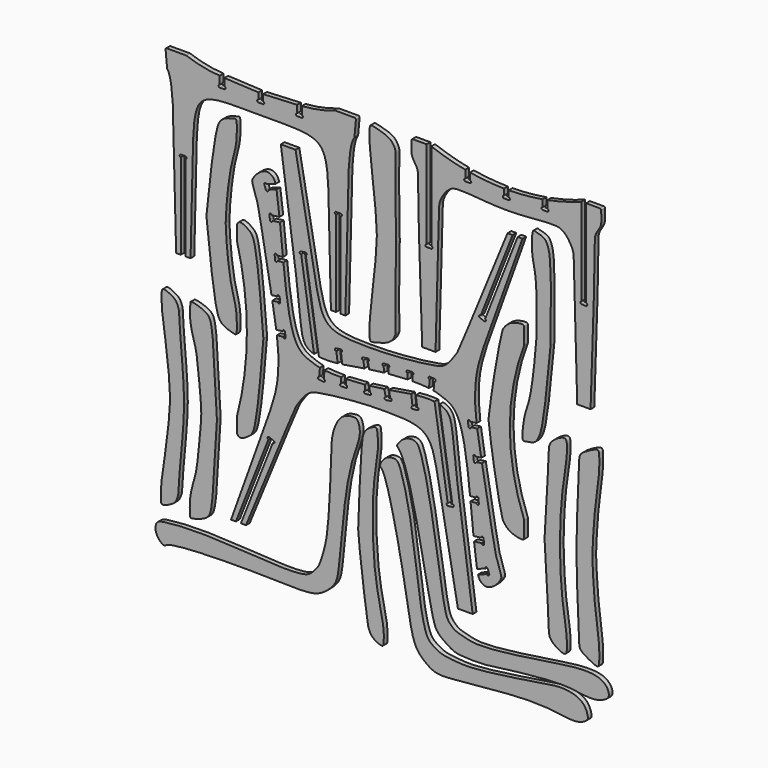
from build123d import *

# Parameters (mm, degrees)
F1_DEPTH = 11.90625
F3_DEPTH = 11.90625
F5_DEPTH = 11.90625
F7_DEPTH = 11.90625


with BuildPart() as f1:
    # F0 (on Front) → F1 (new body)
    with BuildSketch(Plane.XZ):
        with BuildLine():
            Line((-81.6249251366, 184.9817527294), (-81.6249251366, 205.2300572395))
            ThreePointArc((-81.6249251366, 205.2300572395), (-124.8707299183, 211.0284592013), (-166.8653927493, 222.8719971122))
            Line((-166.8653927493, 222.8719971122), (-216.4043151029, 222.8719971122))
            ThreePointArc((-216.4043151029, 222.8719971122), (-218.7506863203, 221.8359611396), (-219.5657662077, 219.4039921424))
            Line((-219.5657662077, 219.4039921424), (-215.716868639, 177.8753399849))
            add(Edge.make_bspline(
                [(-201.2570202351, 103.3167913556), (-203.5053147842, 133.6572504695), (-205.7536093334, 163.9977095834), (-215.716868639, 177.8753399849)],
                knots=[0, 0, 0, 0, 0.6286084073, 0.6286084073, 0.6286084073, 0.6286084073], degree=3))
            Line((-201.2570202351, 103.3167913556), (-192.6272958517, -229.0771717804))
            Line((-192.6272958517, -229.0771717804), (-180.7148461342, -228.9787826776))
            Line((-180.7148461342, -228.9787826776), (-180.7148461342, -10.1681035912))
            ThreePointArc((-180.7148461342, -10.1681035912), (-183.8898461342, -6.9931035912), (-180.7148461342, -3.8181035912))
            Line((-180.7148461342, -3.8181035912), (-168.8085961342, -3.8181035912))
            ThreePointArc((-168.8085961342, -3.8181035912), (-165.6335961342, -6.9931035912), (-168.8085961342, -10.1681035912))
            Line((-168.8085961342, -10.1681035912), (-168.8085961342, -228.8804447805))
            Line((-168.8085961342, -228.8804447805), (-155.8824628592, -228.7736833096))
            Line((-155.8824628592, -228.7736833096), (-149.3858247995, 40.4817350209))
            add(Edge.make_bspline(
                [(-149.3858247995, 40.4817350209), (-147.4859416485, 69.7398781776), (-146.2123086991, 156.4636002304), (-66.5898651674, 150.1531891202), (23.0572682768, 150.2735537717)],
                knots=[0, 0, 0, 0, 0.4228498511, 0.9834705051, 0.9834705051, 0.9834705051, 0.9834705051], degree=3))
            add(Edge.make_bspline(
                [(195.5003613532, 40.4817350209), (193.6004782021, 69.7398781776), (192.3268452527, 156.4636002304), (112.704401721, 150.1531891202), (23.0572682768, 150.2735537717)],
                knots=[0, 0, 0, 0, 0.4228498511, 0.9834705051, 0.9834705051, 0.9834705051, 0.9834705051], degree=3))
            Line((195.5003613532, 40.4817350209), (201.9969994128, -228.7736833096))
            Line((201.9969994128, -228.7736833096), (214.9231326878, -228.8804447805))
            Line((214.9231326878, -228.8804447805), (214.9231326878, -10.1681035912))
            ThreePointArc((214.9231326878, -10.1681035912), (211.7481326878, -6.9931035912), (214.9231326878, -3.8181035912))
            Line((214.9231326878, -3.8181035912), (226.8293826878, -3.8181035912))
            ThreePointArc((226.8293826878, -3.8181035912), (230.0043826878, -6.9931035912), (226.8293826878, -10.1681035912))
            Line((226.8293826878, -10.1681035912), (226.8293826878, -228.9787826776))
            Line((226.8293826878, -228.9787826776), (238.7418324053, -229.0771717804))
            Line((238.7418324053, -229.0771717804), (247.3715567887, 103.3167913556))
            add(Edge.make_bspline(
                [(247.3715567887, 103.3167913556), (249.6198513379, 133.6572504695), (251.868145887, 163.9977095834), (261.8314051926, 177.8753399849)],
                knots=[0, 0, 0, 0, 0.6286084073, 0.6286084073, 0.6286084073, 0.6286084073], degree=3))
            Line((261.8314051926, 177.8753399849), (265.6803027613, 219.4039921424))
            ThreePointArc((265.6803027613, 219.4039921424), (264.8652228739, 221.8359611396), (262.5188516565, 222.8719971122))
            Line((262.5188516565, 222.8719971122), (212.9799293029, 222.8719971122))
            ThreePointArc((212.9799293029, 222.8719971122), (170.9852664719, 211.0284592013), (127.7394616902, 205.2300572395))
            Line((127.7394616902, 205.2300572395), (127.7394616902, 184.9817527294))
            ThreePointArc((127.7394616902, 184.9817527294), (130.9144616902, 181.8067527294), (127.7394616902, 178.6317527294))
            Line((127.7394616902, 178.6317527294), (115.8332116902, 178.6317527294))
            ThreePointArc((115.8332116902, 178.6317527294), (112.6582116902, 181.8067527294), (115.8332116902, 184.9817527294))
            Line((115.8332116902, 184.9817527294), (115.8332116902, 204.0726095438))
            Line((115.8332116902, 204.0726095438), (29.0103932768, 199.9165117741))
            Line((29.0103932768, 199.9165117741), (29.0103932768, 183.5399461746))
            ThreePointArc((29.0103932768, 183.5399461746), (32.1853932768, 180.3649461746), (29.0103932768, 177.1899461746))
            Line((29.0103932768, 177.1899461746), (23.0572682768, 177.1899461746))
            Line((23.0572682768, 177.1899461746), (17.1041432768, 177.1899461746))
            ThreePointArc((17.1041432768, 177.1899461746), (13.9291432768, 180.3649461746), (17.1041432768, 183.5399461746))
            Line((17.1041432768, 183.5399461746), (17.1041432768, 199.9165117741))
            Line((17.1041432768, 199.9165117741), (-69.7186751366, 204.0726095438))
            Line((-69.7186751366, 204.0726095438), (-69.7186751366, 184.9817527294))
            ThreePointArc((-69.7186751366, 184.9817527294), (-66.5436751366, 181.8067527294), (-69.7186751366, 178.6317527294))
            Line((-69.7186751366, 178.6317527294), (-81.6249251366, 178.6317527294))
            ThreePointArc((-81.6249251366, 178.6317527294), (-84.7999251366, 181.8067527294), (-81.6249251366, 184.9817527294))
        make_face()
    extrude(amount=F1_DEPTH)


with BuildPart() as f1b:
    # F0 (on Front) → F1, piece 2 (new body)
    with BuildSketch(Plane.XZ):
        with BuildLine():
            Line((753.9582689397, 197.8409755017), (753.9392547607, 177.9192579746))
            ThreePointArc((753.9392547607, 177.9192579746), (757.1142547607, 174.7442579746), (753.9392547607, 171.5692579746))
            Line((753.9392547607, 171.5692579746), (742.0330047607, 171.5692579746))
            ThreePointArc((742.0330047607, 171.5692579746), (738.8580047607, 174.7442579746), (742.0330047607, 177.9192579746))
            Line((742.0330047607, 177.9192579746), (742.0330047607, 195.6590753576))
            ThreePointArc((742.0330047607, 195.6590753576), (698.8370899175, 189.9852566287), (655.3285871628, 187.7292721077))
            Line((655.3285871628, 187.7292721077), (655.3285871628, 171.9064457408))
            ThreePointArc((655.3285871628, 171.9064457408), (658.5035871628, 168.7314457408), (655.3285871628, 165.5564457408))
            Line((655.3285871628, 165.5564457408), (649.375430584, 165.5564457408))
            Line((649.375430584, 165.5564457408), (643.4222740051, 165.5564457408))
            ThreePointArc((643.4222740051, 165.5564457408), (640.2472740051, 168.7314457408), (643.4222740051, 171.9064457408))
            Line((643.4222740051, 171.9064457408), (643.4222740051, 187.7292721077))
            ThreePointArc((643.4222740051, 187.7292721077), (599.9137712504, 189.9852566287), (556.7178564072, 195.6590753576))
            Line((556.7178564072, 195.6590753576), (556.7178564072, 177.9192579746))
            ThreePointArc((556.7178564072, 177.9192579746), (559.8928564072, 174.7442579746), (556.7178564072, 171.5692579746))
            Line((556.7178564072, 171.5692579746), (544.8116064072, 171.5692579746))
            ThreePointArc((544.8116064072, 171.5692579746), (541.6366064072, 174.7442579746), (544.8116064072, 177.9192579746))
            Line((544.8116064072, 177.9192579746), (544.7925922282, 197.8409755017))
            ThreePointArc((544.7925922282, 197.8409755017), (500.8902250493, 208.2467794905), (457.9821969142, 222.1966799246))
            Line((457.9821969142, 222.1966799246), (457.8196128837, -1.4435426646))
            ThreePointArc((457.8196128837, -1.4435426646), (460.9842648937, -4.6208339943), (457.8149965181, -7.7935206322))
            Line((457.8149965181, -7.7935206322), (445.9087465181, -7.7935218998))
            ThreePointArc((445.9087465181, -7.7935218998), (442.7744985153, -4.5708815102), (446.0045408796, -1.4442622579))
            Line((446.0045408796, -1.4442622579), (446.0045408796, 222.833275795))
            Line((446.0045408796, 222.833275795), (410.7614188056, 222.833275795))
            ThreePointArc((410.7614188056, 222.833275795), (408.5663096829, 221.9522071234), (407.5894946571, 219.7979976465))
            add(Edge.make_bspline(
                [(407.5894946571, 219.7979976465), (407.0855216225, 208.3569508739), (406.4295588438, 189.5758183878), (411.4862805096, 177.3822155111), (425.682188243, 158.4107209843), (422.6201017336, 109.1856224555), (429.5663710054, -88.2138828921), (434.7653226852, -235.9580099583)],
                knots=[0.0119439068, 0.0119439068, 0.0119439068, 0.0119439068, 0.1472174846, 0.2400583983, 0.3538051352, 0.5163539238, 1, 1, 1, 1], degree=3))
            Line((434.7653226852, -235.9580099583), (468.7381820679, -235.9580099583))
            add(Edge.make_bspline(
                [(468.7381820679, -235.9580099583), (472.4303966062, -104.6167901897), (477.3449907849, 70.2075022277), (477.7680787876, 108.7569713641), (502.1370780301, 143.5053595047), (529.180974636, 149.9698487576), (609.7624332079, 141.4228850822), (638.3718253047, 141.2618428968), (649.3754305839, 141.2687947189)],
                knots=[0, 0, 0, 0, 0.3522357263, 0.4688502339, 0.5878047938, 0.6920991895, 0.8721155501, 0.9906857663, 0.9906857663, 0.9906857663, 0.9906857663], degree=3))
            add(Edge.make_bspline(
                [(830.0126791, -235.9580099583), (826.3204645618, -104.6167901897), (821.405870383, 70.2075022277), (820.9827823803, 108.7569713641), (796.6137831378, 143.5053595047), (769.5698865319, 149.9698487576), (688.98842796, 141.4228850822), (660.3790358632, 141.2618428968), (649.3754305839, 141.2687947189)],
                knots=[0, 0, 0, 0, 0.3522357263, 0.4688502339, 0.5878047938, 0.6920991895, 0.8721155501, 0.9906857663, 0.9906857663, 0.9906857663, 0.9906857663], degree=3))
            Line((830.0126791, -235.9580099583), (863.9855384827, -235.9580099583))
            add(Edge.make_bspline(
                [(891.1613665108, 219.7979976465), (891.6653395454, 208.3569508739), (892.3213023241, 189.5758183878), (887.2645806583, 177.3822155111), (873.0686729249, 158.4107209843), (876.1307594343, 109.1856224555), (869.1844901625, -88.2138828921), (863.9855384827, -235.9580099583)],
                knots=[0.0119439068, 0.0119439068, 0.0119439068, 0.0119439068, 0.1472174846, 0.2400583983, 0.3538051352, 0.5163539238, 1, 1, 1, 1], degree=3))
            ThreePointArc((891.1613665108, 219.7979976465), (890.184551485, 221.9522071234), (887.9894423623, 222.833275795))
            Line((887.9894423623, 222.833275795), (852.7463202883, 222.833275795))
            Line((852.7463202883, 222.833275795), (852.7463202883, -1.4442622579))
            ThreePointArc((852.7463202883, -1.4442622579), (855.9763626526, -4.5708815102), (852.8421146498, -7.7935218998))
            Line((852.8421146498, -7.7935218998), (840.9358646498, -7.7935206322))
            ThreePointArc((840.9358646498, -7.7935206322), (837.7665962742, -4.6208339943), (840.9312482842, -1.4435426646))
            Line((840.9312482842, -1.4435426646), (840.7686642537, 222.1966799246))
            ThreePointArc((840.7686642537, 222.1966799246), (797.8606361186, 208.2467794905), (753.9582689397, 197.8409755017))
        make_face()
    extrude(amount=F1_DEPTH)


with BuildPart() as f3:
    # F2 (on Front) → F3 (new body)
    with BuildSketch(Plane.XZ):
        with BuildLine():
            add(Edge.make_bspline(
                [(566.8695082514, -629.2812363074), (569.5853295665, -654.3702688331), (572.1095143597, -675.1237511334), (574.4261674133, -688.4633543022)],
                knots=[0.5041739496, 0.5041739496, 0.5041739496, 0.5041739496, 0.5323722078, 0.5323722078, 0.5323722078, 0.5323722078], degree=3))
            Line((574.4261674133, -688.4633543022), (595.5900230834, -680.886998067))
            ThreePointArc((595.5900230834, -680.886998067), (597.509152839, -676.827664257), (601.568486649, -678.7467940126))
            Line((601.568486649, -678.7467940126), (605.581369251, -689.9564131981))
            ThreePointArc((605.581369251, -689.9564131981), (603.6622394954, -694.0157470081), (599.6029056854, -692.0966172525))
            Line((599.6029056854, -692.0966172525), (576.9251566248, -700.2149255691))
            add(Edge.make_bspline(
                [(576.9251566248, -700.2149255691), (577.9995338219, -704.1085984084), (580.5037674854, -710.1106761836), (586.6774372848, -717.4303434775), (600.064292499, -722.9901001137), (619.8937899939, -713.2743570691), (632.3782583366, -697.6701022409), (639.353554629, -686.8491619857), (623.0185314321, -652.1785312949), (612.0860881001, -584.9638273352), (595.1931225708, -492.5807100816), (587.236787797, -447.3290557083)],
                knots=[0.5426631517, 0.5426631517, 0.5426631517, 0.5426631517, 0.5556846822, 0.5709687245, 0.5884954803, 0.6108677295, 0.6326246328, 0.6485941027, 0.6762818943, 0.7187139825, 0.7710183017, 0.7710183017, 0.7710183017, 0.7710183017], degree=3))
            Line((587.236787797, -447.3290557084), (572.6997915784, -449.1565687147))
            ThreePointArc((572.6997915784, -449.1565687147), (569.9456139325, -452.7027998824), (566.3993827648, -449.9486222365))
            Line((566.3993827648, -449.9486222365), (564.9142824113, -438.135355711))
            ThreePointArc((564.9142824113, -438.135355711), (567.6684600572, -434.5891245433), (571.2146912249, -437.3433021891))
            Line((571.2146912249, -437.3433021891), (585.1811060506, -435.5875196078))
            add(Edge.make_bspline(
                [(585.1811060506, -435.5875196079), (584.4323143041, -431.2907071066), (580.526436641, -408.7505367433), (577.1870397166, -388.6642774653), (575.0108794965, -373.3527850809)],
                knots=[0.775597785, 0.775597785, 0.775597785, 0.775597785, 0.7806933084, 0.8027679956, 0.8027679956, 0.8027679956, 0.8027679956], degree=3))
            Line((575.0108794965, -373.3527850808), (559.0072337667, -375.3646773782))
            ThreePointArc((559.0072337667, -375.3646773782), (556.2530561208, -378.9109085459), (552.706824953, -376.1567309001))
            Line((552.706824953, -376.1567309001), (551.2217245996, -364.3434643745))
            ThreePointArc((551.2217245996, -364.3434643745), (553.9759022455, -360.7972332068), (557.5221334132, -363.5514108527))
            Line((557.5221334132, -363.5514108527), (573.4188186259, -361.5529650564))
            add(Edge.make_bspline(
                [(573.4188186259, -361.5529650565), (571.541615983, -346.7842885987), (567.7068869039, -305.7710886357), (572.2446272444, -236.4022129148), (605.6116131937, -145.0539413696), (673.6225943328, 43.7902893513), (690.3986930847, 90.3371274471)],
                knots=[0.8085324624, 0.8085324624, 0.8085324624, 0.8085324624, 0.8305204676, 0.8732825465, 0.9238130436, 1, 1, 1, 1], degree=3))
            Line((690.3986930847, 90.3371274471), (677.9750958085, 90.3371274471))
            Line((677.9750958085, 90.3371274471), (595.1901786029, -120.6226050854))
            ThreePointArc((595.1901786029, -120.6226050854), (596.9859254868, -124.7380082405), (592.8705223316, -126.5337551243))
            Line((592.8705223316, -126.5337551243), (581.7871160086, -122.1843996156))
            ThreePointArc((581.7871160086, -122.1843996156), (579.9913691248, -118.0689964605), (584.1067722799, -116.2732495767))
            Line((584.1067722799, -116.2732495767), (665.1849133564, 90.3371274471))
            Line((665.1849133564, 90.3371274471), (652.2805280983, 90.3371274471))
            add(Edge.make_bspline(
                [(652.2805280983, 90.3371274471), (596.7992489646, -44.9195170026), (529.8230377107, -208.1994148996), (523.2153969383, -221.3143134207), (497.4125593379, -258.4004771389), (467.6212718132, -269.0955724434), (359.0838115877, -280.6103699551), (283.1255249355, -281.2402915833), (222.7475667298, -278.8147196555), (191.4119530649, -263.556681825), (172.6586255781, -230.6504371588), (157.6041323146, -145.7013190048), (129.7748164105, 4.8959686394), (111.855674535, 101.8647253513)],
                knots=[0, 0, 0, 0, 0.1855154705, 0.2239516381, 0.2883693718, 0.3471684711, 0.4532029351, 0.5467207513, 0.6247930511, 0.6828197717, 0.7416883994, 0.8336745957, 1, 1, 1, 1], degree=3))
            Line((111.855674535, 101.8647253513), (74.2674358189, 101.8647253513))
            add(Edge.make_bspline(
                [(74.2674358189, 101.8647253513), (78.8915198201, 69.5147677357), (83.5137174572, 37.1780070688), (87.9711113313, 5.7144869035)],
                knots=[0, 0, 0, 0, 0.0229430236, 0.0229430236, 0.0229430236, 0.0229430236], degree=3))
            add(Edge.make_bspline(
                [(87.9711113313, 5.7144869035), (100.6031911897, -83.4518983389), (119.6075895959, -221.5137269482), (125.5186145516, -299.1595751985), (134.8803023203, -330.0648259095), (149.5395161253, -338.7788583075), (158.9980423115, -341.3134779083)],
                knots=[0.0229430236, 0.0229430236, 0.0229430236, 0.0229430236, 0.0879626549, 0.1322113205, 0.1576764492, 0.1813971108, 0.1813971108, 0.1813971108, 0.1813971108], degree=3))
            Line((158.9980423115, -341.3134779083), (126.1187144879, -128.2851324575))
            ThreePointArc((126.1187144879, -128.2851324575), (122.4965658301, -125.6315897123), (125.1501085753, -122.0094410544))
            Line((125.1501085753, -122.0094410544), (136.917029956, -120.1933049683))
            ThreePointArc((136.917029956, -120.1933049683), (140.5391786138, -122.8468477135), (137.8856358686, -126.4689963713))
            Line((137.8856358686, -126.4689963713), (171.394359373, -343.5752573204))
            add(Edge.make_bspline(
                [(171.394359373, -343.5752573204), (184.8736689285, -345.1120254544), (201.6749889802, -344.5009932843), (218.5750232266, -342.6842309365), (219.1755757519, -342.6182161686)],
                knots=[0.1908558182, 0.1908558182, 0.1908558182, 0.1908558182, 0.2194262024, 0.2204785746, 0.2204785746, 0.2204785746, 0.2204785746], degree=3))
            Line((219.1755757519, -342.6182161686), (215.869193574, -316.3175195105))
            ThreePointArc((215.869193574, -316.3175195105), (212.3229624062, -313.5633418646), (215.0771400521, -310.0171106969))
            Line((215.0771400521, -310.0171106969), (226.8904065776, -308.5320103434))
            ThreePointArc((226.8904065776, -308.5320103434), (230.4366377453, -311.2861879893), (227.6824600995, -314.832419157))
            Line((227.6824600995, -314.832419157), (230.9906811714, -341.1477433423))
            add(Edge.make_bspline(
                [(230.9906811715, -341.1477433423), (249.07955335, -338.6582784106), (267.5544694031, -335.1362268397), (287.5048138783, -331.8922872279)],
                knots=[0.2273609107, 0.2273609107, 0.2273609107, 0.2273609107, 0.2588542647, 0.2588542647, 0.2588542647, 0.2588542647], degree=3))
            Line((287.5048138784, -331.8922872279), (284.5437138697, -314.7883116116))
            ThreePointArc((284.5437138697, -314.7883116116), (280.8736399921, -312.2014587489), (283.4604928548, -308.5313848714))
            Line((283.4604928548, -308.5313848714), (295.1922304928, -306.5003454685))
            ThreePointArc((295.1922304928, -306.5003454685), (298.8623043704, -309.0871983312), (296.2754515077, -312.7572722088))
            Line((296.2754515077, -312.7572722088), (299.2688604156, -330.0478712496))
            add(Edge.make_bspline(
                [(299.2688604156, -330.0478712496), (311.6334559032, -328.1866698123), (324.5238565238, -326.4939882328), (337.5390271034, -325.0741291087)],
                knots=[0.2649537217, 0.2649537217, 0.2649537217, 0.2649537217, 0.2839083997, 0.2839083997, 0.2839083997, 0.2839083997], degree=3))
            Line((337.5390271034, -325.0741291087), (336.3677488719, -310.9681260445))
            ThreePointArc((336.3677488719, -310.9681260445), (332.9409089755, -308.0667439041), (335.8422911159, -304.6399040078))
            Line((335.8422911159, -304.6399040078), (347.7077074349, -303.6546707153))
            ThreePointArc((347.7077074349, -303.6546707153), (351.1345473313, -306.5560528557), (348.2331651908, -309.9828927521))
            Line((348.2331651908, -309.9828927521), (349.3856222375, -323.8622274778))
            add(Edge.make_bspline(
                [(349.3856222375, -323.8622274778), (363.9828662923, -322.4699635009), (380.41617949, -321.3314170465), (396.1444916825, -320.8597404872), (397.8871803284, -320.8154072931)],
                knots=[0.2896480836, 0.2896480836, 0.2896480836, 0.2896480836, 0.3108436467, 0.313502856, 0.313502856, 0.313502856, 0.313502856], degree=3))
            Line((397.8871803284, -320.8154072931), (397.4540628227, -307.0115702828))
            ThreePointArc((397.4540628227, -307.0115702828), (394.1810528385, -303.9377037205), (397.2549194007, -300.6646937362))
            Line((397.2549194007, -300.6646937362), (409.1553129256, -300.2912998199))
            ThreePointArc((409.1553129256, -300.2912998199), (412.4283229099, -303.3651663822), (409.3544563476, -306.6381763665))
            Line((409.3544563476, -306.6381763665), (409.7937739849, -320.6396170431))
            add(Edge.make_bspline(
                [(409.793773985, -320.6396170431), (425.7267691669, -320.5793075671), (440.3219423663, -321.2493581383), (451.9999158307, -322.6158233251)],
                knots=[0.3196576333, 0.3196576333, 0.3196576333, 0.3196576333, 0.3448245133, 0.3448245133, 0.3448245133, 0.3448245133], degree=3))
            Line((451.9999158307, -322.6158233251), (453.8983790613, -302.3204325437))
            ThreePointArc((453.8983790613, -302.3204325437), (451.0328829105, -298.8635290436), (454.4897864107, -295.9980328927))
            Line((454.4897864107, -295.9980328927), (466.3442857563, -297.1069216728))
            ThreePointArc((466.3442857563, -297.1069216728), (469.2097819072, -300.563825173), (465.752878407, -303.4293213238))
            Line((465.752878407, -303.4293213238), (463.7880346946, -324.4343480869))
            add(Edge.make_bspline(
                [(463.7880346946, -324.4343480869), (471.9039207593, -326.0572697828), (487.0014775824, -331.2603228654), (536.9638470038, -348.6264520909), (549.6036944238, -459.5964349534), (556.7808309902, -530.3787318412)],
                knots=[0.3542148453, 0.3542148453, 0.3542148453, 0.3542148453, 0.3759368259, 0.4073734484, 0.4717986423, 0.4717986423, 0.4717986423, 0.4717986423], degree=3))
            Line((556.7808309902, -530.3787318412), (571.8823122062, -529.2545845291))
            ThreePointArc((571.8823122062, -529.2545845291), (574.8128584467, -525.8526514415), (578.2147915343, -528.7831976821))
            Line((578.2147915343, -528.7831976821), (579.0986418724, -540.6565964222))
            ThreePointArc((579.0986418724, -540.6565964222), (576.1680956319, -544.0585295097), (572.7661625443, -541.1279832692))
            Line((572.7661625443, -541.1279832692), (557.9763695577, -542.228928653))
            add(Edge.make_bspline(
                [(557.9763695577, -542.228928653), (560.6548814033, -568.8653653623), (563.2016059701, -594.6039142121), (565.6061929157, -617.4400881619)],
                knots=[0.4754072925, 0.4754072925, 0.4754072925, 0.4754072925, 0.4998482581, 0.4998482581, 0.4998482581, 0.4998482581], degree=3))
            Line((565.6061929158, -617.4400881619), (584.813059481, -615.0255041632))
            ThreePointArc((584.813059481, -615.0255041632), (587.5672371269, -611.4792729955), (591.1134682947, -614.2334506414))
            Line((591.1134682947, -614.2334506414), (592.5985686481, -626.0467171669))
            ThreePointArc((592.5985686481, -626.0467171669), (589.8443910022, -629.5929483346), (586.2981598345, -626.8387706887))
            Line((586.2981598345, -626.8387706887), (566.8695082514, -629.2812363074))
        make_face()
    extrude(amount=F3_DEPTH)


with BuildPart() as f3b:
    # F2 (on Front) → F3, piece 2 (new body)
    with BuildSketch(Plane.XZ):
        with BuildLine():
            Line((525.8545875549, -793.4511899948), (563.4428262711, -793.4511899948))
            add(Edge.make_bspline(
                [(563.4428262711, -793.4511899948), (558.8187422699, -761.1012323792), (554.1965446328, -728.7644717123), (549.7391507587, -697.300951547)],
                knots=[0, 0, 0, 0, 0.0229430236, 0.0229430236, 0.0229430236, 0.0229430236], degree=3))
            add(Edge.make_bspline(
                [(549.7391507587, -697.300951547), (537.1070709003, -608.1345663045), (518.1026724941, -470.0727376953), (512.1916475384, -392.4268894449), (502.8299597697, -361.521638734), (488.1707459647, -352.807606336), (478.7122197784, -350.2729867352)],
                knots=[0.0229430236, 0.0229430236, 0.0229430236, 0.0229430236, 0.0879626549, 0.1322113205, 0.1576764492, 0.1813971108, 0.1813971108, 0.1813971108, 0.1813971108], degree=3))
            Line((478.7122197784, -350.2729867352), (511.591547602, -563.301332186))
            ThreePointArc((511.591547602, -563.301332186), (515.2136962599, -565.9548749312), (512.5601535147, -569.577023589))
            Line((512.5601535147, -569.577023589), (500.793232134, -571.3931596752))
            ThreePointArc((500.793232134, -571.3931596752), (497.1710834762, -568.73961693), (499.8246262214, -565.1174682722))
            Line((499.8246262214, -565.1174682722), (466.315902717, -348.0112073231))
            add(Edge.make_bspline(
                [(466.315902717, -348.0112073231), (452.8365931615, -346.4744391891), (436.0352731098, -347.0854713592), (419.1352388633, -348.902233707), (418.5346863381, -348.9682484749)],
                knots=[0.1908558182, 0.1908558182, 0.1908558182, 0.1908558182, 0.2194262024, 0.2204785746, 0.2204785746, 0.2204785746, 0.2204785746], degree=3))
            Line((418.5346863381, -348.9682484749), (421.841068516, -375.268945133))
            ThreePointArc((421.841068516, -375.268945133), (425.3872996837, -378.0231227789), (422.6331220379, -381.5693539466))
            Line((422.6331220379, -381.5693539466), (410.8198555123, -383.0544543001))
            ThreePointArc((410.8198555123, -383.0544543001), (407.2736243446, -380.3002766542), (410.0278019905, -376.7540454865))
            Line((410.0278019905, -376.7540454865), (406.7195809185, -350.4387213011))
            add(Edge.make_bspline(
                [(406.7195809185, -350.4387213011), (388.63070874, -352.9281862329), (370.1557926869, -356.4502378038), (350.2054482116, -359.6941774156)],
                knots=[0.2273609107, 0.2273609107, 0.2273609107, 0.2273609107, 0.2588542647, 0.2588542647, 0.2588542647, 0.2588542647], degree=3))
            Line((350.2054482116, -359.6941774156), (353.1665482203, -376.7981530319))
            ThreePointArc((353.1665482203, -376.7981530319), (356.8366220978, -379.3850058946), (354.2497692351, -383.0550797721))
            Line((354.2497692351, -383.0550797721), (342.5180315971, -385.086119175))
            ThreePointArc((342.5180315971, -385.086119175), (338.8479577196, -382.4992663123), (341.4348105823, -378.8291924347))
            Line((341.4348105823, -378.8291924347), (338.4414016744, -361.5385933939))
            add(Edge.make_bspline(
                [(338.4414016744, -361.5385933939), (326.0768061867, -363.3997948312), (313.1864055661, -365.0924764106), (300.1712349866, -366.5123355348)],
                knots=[0.2649537217, 0.2649537217, 0.2649537217, 0.2649537217, 0.2839083997, 0.2839083997, 0.2839083997, 0.2839083997], degree=3))
            Line((300.1712349866, -366.5123355348), (301.3425132181, -380.618338599))
            ThreePointArc((301.3425132181, -380.618338599), (304.7693531144, -383.5197207394), (301.867970974, -386.9465606357))
            Line((301.867970974, -386.9465606357), (290.0025546551, -387.9317939281))
            ThreePointArc((290.0025546551, -387.9317939281), (286.5757147587, -385.0304117877), (289.4770968991, -381.6035718914))
            Line((289.4770968991, -381.6035718914), (288.3246398525, -367.7242371657))
            add(Edge.make_bspline(
                [(288.3246398525, -367.7242371657), (273.7273957977, -369.1165011426), (257.2940825999, -370.255047597), (241.5657704075, -370.7267241563), (239.8230817615, -370.7710573503)],
                knots=[0.2896480836, 0.2896480836, 0.2896480836, 0.2896480836, 0.3108436467, 0.313502856, 0.313502856, 0.313502856, 0.313502856], degree=3))
            Line((239.8230817615, -370.7710573503), (240.2561992672, -384.5748943607))
            ThreePointArc((240.2561992672, -384.5748943607), (243.5292092515, -387.648760923), (240.4553426892, -390.9217709073))
            Line((240.4553426892, -390.9217709073), (228.5549491644, -391.2951648235))
            ThreePointArc((228.5549491644, -391.2951648235), (225.2819391801, -388.2212982612), (228.3558057424, -384.948288277))
            Line((228.3558057424, -384.948288277), (227.916488105, -370.9468476004))
            add(Edge.make_bspline(
                [(227.916488105, -370.9468476004), (211.9834929231, -371.0071570764), (197.3883197237, -370.3371065052), (185.7103462593, -368.9706413184)],
                knots=[0.3196576333, 0.3196576333, 0.3196576333, 0.3196576333, 0.3448245133, 0.3448245133, 0.3448245133, 0.3448245133], degree=3))
            Line((185.7103462592, -368.9706413184), (183.8118830286, -389.2660320997))
            ThreePointArc((183.8118830286, -389.2660320997), (186.6773791795, -392.7229355999), (183.2204756793, -395.5884317507))
            Line((183.2204756793, -395.5884317507), (171.3659763336, -394.4795429707))
            ThreePointArc((171.3659763336, -394.4795429707), (168.5004801828, -391.0226394705), (171.957383683, -388.1571433196))
            Line((171.957383683, -388.1571433196), (173.9222273954, -367.1521165565))
            add(Edge.make_bspline(
                [(173.9222273954, -367.1521165565), (165.8063413306, -365.5291948606), (150.7087845075, -360.3261417781), (100.7464150861, -342.9600125526), (88.1065676661, -231.99002969), (80.9294310997, -161.2077328022)],
                knots=[0.3542148453, 0.3542148453, 0.3542148453, 0.3542148453, 0.3759368259, 0.4073734484, 0.4717986423, 0.4717986423, 0.4717986423, 0.4717986423], degree=3))
            Line((80.9294310997, -161.2077328023), (65.8279498838, -162.3318801144))
            ThreePointArc((65.8279498838, -162.3318801144), (62.8974036433, -165.7338132019), (59.4954705557, -162.8032669614))
            Line((59.4954705557, -162.8032669614), (58.6116202176, -150.9298682213))
            ThreePointArc((58.6116202176, -150.9298682213), (61.5421664581, -147.5279351337), (64.9440995456, -150.4584813743))
            Line((64.9440995456, -150.4584813743), (79.7338925323, -149.3575359905))
            add(Edge.make_bspline(
                [(79.7338925323, -149.3575359905), (77.0553806866, -122.7210992812), (74.5086561198, -96.9825504313), (72.1040691742, -74.1463764816)],
                knots=[0.4754072925, 0.4754072925, 0.4754072925, 0.4754072925, 0.4998482581, 0.4998482581, 0.4998482581, 0.4998482581], degree=3))
            Line((72.1040691742, -74.1463764816), (52.8972026089, -76.5609604802))
            ThreePointArc((52.8972026089, -76.5609604802), (50.143024963, -80.107191648), (46.5967937953, -77.3530140021))
            Line((46.5967937953, -77.3530140021), (45.1116934419, -65.5397474766))
            ThreePointArc((45.1116934419, -65.5397474766), (47.8658710878, -61.9935163089), (51.4121022555, -64.7476939547))
            Line((51.4121022555, -64.7476939547), (70.8407538386, -62.305228336))
            add(Edge.make_bspline(
                [(70.8407538385, -62.305228336), (68.1249325235, -37.2161958104), (65.6007477302, -16.4627135101), (63.2840946767, -3.1231103413)],
                knots=[0.5041739496, 0.5041739496, 0.5041739496, 0.5041739496, 0.5323722078, 0.5323722078, 0.5323722078, 0.5323722078], degree=3))
            Line((63.2840946767, -3.1231103413), (42.1202390066, -10.6994665765))
            ThreePointArc((42.1202390066, -10.6994665765), (40.201109251, -14.7588003865), (36.141775441, -12.8396706309))
            Line((36.141775441, -12.8396706309), (32.128892839, -1.6300514454))
            ThreePointArc((32.128892839, -1.6300514454), (34.0480225946, 2.4292823647), (38.1073564046, 0.5101526091))
            Line((38.1073564046, 0.5101526091), (60.7851054652, 8.6284609256))
            add(Edge.make_bspline(
                [(60.7851054652, 8.6284609256), (59.7107282681, 12.5221337649), (57.2064946046, 18.5242115402), (51.0328248052, 25.843878834), (37.645969591, 31.4036354702), (17.8164720961, 21.6878924256), (5.3320037534, 6.0836375974), (-1.643292539, -4.7373026578), (14.6917306579, -39.4079333486), (25.6241739899, -106.6226373082), (42.5171395192, -199.0057545618), (50.473474293, -244.2574089351)],
                knots=[0.5426631517, 0.5426631517, 0.5426631517, 0.5426631517, 0.5556846822, 0.5709687245, 0.5884954803, 0.6108677295, 0.6326246328, 0.6485941027, 0.6762818943, 0.7187139825, 0.7710183017, 0.7710183017, 0.7710183017, 0.7710183017], degree=3))
            Line((50.473474293, -244.2574089351), (65.0104705116, -242.4298959288))
            ThreePointArc((65.0104705116, -242.4298959288), (67.7646481575, -238.8836647611), (71.3108793252, -241.637842407))
            Line((71.3108793252, -241.637842407), (72.7959796786, -253.4511089325))
            ThreePointArc((72.7959796786, -253.4511089325), (70.0418020327, -256.9973401002), (66.495570865, -254.2431624543))
            Line((66.495570865, -254.2431624543), (52.5291560394, -255.9989450356))
            add(Edge.make_bspline(
                [(52.5291560394, -255.9989450356), (53.2779477858, -260.2957575369), (57.183825449, -282.8359279002), (60.5232223734, -302.9221871782), (62.6993825935, -318.2336795626)],
                knots=[0.775597785, 0.775597785, 0.775597785, 0.775597785, 0.7806933084, 0.8027679956, 0.8027679956, 0.8027679956, 0.8027679956], degree=3))
            Line((62.6993825935, -318.2336795627), (78.7030283233, -316.2217872653))
            ThreePointArc((78.7030283233, -316.2217872653), (81.4572059692, -312.6755560975), (85.0034371369, -315.4297337434))
            Line((85.0034371369, -315.4297337434), (86.4885374904, -327.2430002689))
            ThreePointArc((86.4885374904, -327.2430002689), (83.7343598445, -330.7892314367), (80.1881286768, -328.0350537908))
            Line((80.1881286768, -328.0350537908), (64.291443464, -330.033499587))
            add(Edge.make_bspline(
                [(64.291443464, -330.033499587), (66.168646107, -344.8021760448), (70.0033751861, -385.8153760078), (65.4656348456, -455.1842517287), (32.0986488963, -546.5325232738), (-35.9123322428, -735.3767539948), (-52.6884309947, -781.9235920906)],
                knots=[0.8085324624, 0.8085324624, 0.8085324624, 0.8085324624, 0.8305204676, 0.8732825465, 0.9238130436, 1, 1, 1, 1], degree=3))
            Line((-52.6884309947, -781.9235920906), (-40.2648337185, -781.9235920906))
            Line((-40.2648337185, -781.9235920906), (42.520083487, -570.9638595581))
            ThreePointArc((42.520083487, -570.9638595581), (40.7243366032, -566.848456403), (44.8397397583, -565.0527095192))
            Line((44.8397397583, -565.0527095192), (55.9231460814, -569.4020650279))
            ThreePointArc((55.9231460814, -569.4020650279), (57.7188929652, -573.517468183), (53.6034898101, -575.3132150668))
            Line((53.6034898101, -575.3132150668), (-27.4746512664, -781.9235920906))
            Line((-27.4746512664, -781.9235920906), (-14.5702660084, -781.9235920906))
            add(Edge.make_bspline(
                [(-14.5702660084, -781.9235920906), (40.9110131254, -646.6669476409), (107.8872243792, -483.3870497439), (114.4948651517, -470.2721512228), (140.2977027521, -433.1859875046), (170.0889902768, -422.4908922), (278.6264505023, -410.9760946884), (354.5847371545, -410.3461730602), (414.9626953602, -412.7717449879), (446.298309025, -428.0297828184), (465.0516365119, -460.9360274846), (480.1061297754, -545.8851456387), (507.9354456794, -696.4824332828), (525.8545875549, -793.4511899948)],
                knots=[0, 0, 0, 0, 0.1855154705, 0.2239516381, 0.2883693718, 0.3471684711, 0.4532029351, 0.5467207513, 0.6247930511, 0.6828197717, 0.7416883994, 0.8336745957, 1, 1, 1, 1], degree=3))
        make_face()
    extrude(amount=F3_DEPTH)


with BuildPart() as f5:
    # F4 (on Front) → F5 (new body)
    with BuildSketch(Plane.XZ):
        with BuildLine():
            add(Edge.make_bspline(
                [(-185.2634698153, -358.3788573742), (-182.9975650718, -409.959197383), (-173.8162417925, -494.204343153), (-172.6510184968, -543.6857300857), (-172.4079746036, -562.5447261506)],
                knots=[0, 0, 0, 0, 0.593650821, 0.9813998786, 0.9813998786, 0.9813998786, 0.9813998786], degree=3))
            add(Edge.make_bspline(
                [(-185.2634698153, -358.3788573742), (-185.5497568201, -352.5088954968), (-191.338871265, -335.8536585817), (-203.6070918592, -327.9856109503), (-219.7048305902, -319.8704468533), (-227.270700623, -320.3623808126), (-230.9306114085, -327.44384459), (-228.5344805812, -379.6382585976), (-221.3058946656, -420.6300621636), (-210.2077258868, -508.1040987328), (-208.5679560022, -545.0757699545), (-207.9144055828, -562.5575401008)],
                knots=[0, 0, 0, 0, 0.0966104982, 0.177788655, 0.2644177776, 0.3157589375, 0.366162426, 0.5098663397, 0.6527992815, 0.8445905386, 0.9950691749, 0.9950691749, 0.9950691749, 0.9950691749], degree=3))
            add(Edge.make_bspline(
                [(-187.1091477657, -767.0328913138), (-187.4418322152, -772.9128691368), (-193.3594694057, -789.5053176296), (-205.6889397905, -797.2836458735), (-221.8492381957, -805.2719409717), (-229.4111842742, -804.7208465411), (-233.0152178925, -797.6136330043), (-230.2197962914, -745.4103189186), (-222.6391353301, -704.6138172548), (-210.947620998, -616.1142599295), (-208.7175518994, -580.4664051973), (-207.9144055828, -562.5575401008)],
                knots=[0, 0, 0, 0, 0.0968150436, 0.1781650722, 0.2649776074, 0.3164274677, 0.3669376713, 0.5109458374, 0.6541813992, 0.84637872, 0.999854206, 0.999854206, 0.999854206, 0.999854206], degree=3))
            add(Edge.make_bspline(
                [(-187.1091477657, -767.0328913138), (-184.4228245705, -715.1067121537), (-174.6632304011, -629.4083577428), (-172.792718331, -582.0441010495), (-172.4079746036, -562.5447261506)],
                knots=[0, 0, 0, 0, 0.5978537767, 1, 1, 1, 1], degree=3))
        make_face()
    extrude(amount=F5_DEPTH)


with BuildPart() as f5b:
    # F4 (on Front) → F5, piece 2 (new body)
    with BuildSketch(Plane.XZ):
        with BuildLine():
            add(Edge.make_bspline(
                [(-88.6324346066, -569.3273544312), (-92.1748193671, -624.0095913029), (-96.8163376082, -712.9088913745), (-101.85992608, -772.6337879095), (-109.6605297773, -796.5477334562), (-130.526593567, -806.3202323355), (-155.8866939916, -813.1805755208), (-157.673608268, -806.7553142819), (-159.7790756763, -758.3661619984), (-140.5252463143, -710.0978207187), (-135.3539050595, -646.7235941547), (-129.1415194025, -594.3526600967), (-128.4593492746, -568.4091448784)],
                knots=[0, 0, 0, 0, 0.1826085112, 0.2950327404, 0.3640026768, 0.4363795428, 0.508609216, 0.5379361089, 0.6377831332, 0.7486408767, 0.8670222861, 1, 1, 1, 1], degree=3))
            add(Edge.make_bspline(
                [(-88.6324346066, -569.3273544312), (-92.0554913448, -514.3850031409), (-96.3013815865, -423.9854856431), (-101.2591687453, -364.3411807666), (-108.9943522492, -340.3736879868), (-129.8377404098, -330.557754133), (-155.1803988462, -323.6329070587), (-156.9834179998, -330.0540049997), (-159.2058399907, -378.4376961216), (-140.0832038069, -426.7532966996), (-135.0189737489, -490.1305429455), (-129.0766090729, -542.5002930017), (-128.4593492746, -568.4091448784)],
                knots=[0, 0, 0, 0, 0.183448372, 0.2957651772, 0.3646692113, 0.4369769195, 0.5091375755, 0.538436446, 0.6381880641, 0.7489398805, 0.8672081737, 1, 1, 1, 1], degree=3))
        make_face()
    extrude(amount=F5_DEPTH)


with BuildPart() as f5c:
    # F4 (on Front) → F5, piece 3 (new body)
    with BuildSketch(Plane.XZ):
        with BuildLine():
            add(Edge.make_bspline(
                [(-115.5187136748, -120.4398870467), (-103.9435007391, -8.1283692628), (-94.2071460134, 66.1345712245), (-83.3728218348, 102.634018771), (-68.9442323432, 114.6997011318), (-48.268468785, 120.4343729614), (-40.482614594, 122.3678238637), (-37.3747364721, 116.7846203024), (-37.030516538, 63.9064810889), (-52.1760649177, 23.9864245776), (-63.2221348379, -56.031678412), (-65.8915948056, -106.8272707669), (-66.3303794613, -120.4398870468)],
                knots=[0.0053428848, 0.0053428848, 0.0053428848, 0.0053428848, 0.2212165437, 0.3010629606, 0.365617231, 0.4370188325, 0.4765335177, 0.5080224641, 0.614995533, 0.7206745161, 0.8714107217, 0.9485925678, 0.9485925678, 0.9485925678, 0.9485925678], degree=3))
            add(Edge.make_bspline(
                [(-115.5187136748, -120.4398870467), (-103.9435007392, -232.7514048307), (-94.2071460134, -307.0143453181), (-83.3728218348, -343.5137928646), (-68.9442323432, -355.5794752254), (-48.268468785, -361.314147055), (-40.482614594, -363.2475979573), (-37.3747364721, -357.664394396), (-37.030516538, -304.7862551826), (-52.1760649177, -264.8661986713), (-63.2221348379, -184.8480956816), (-65.8915948056, -134.0525033267), (-66.3303794613, -120.4398870468)],
                knots=[0.0053428848, 0.0053428848, 0.0053428848, 0.0053428848, 0.2212165437, 0.3010629606, 0.365617231, 0.4370188325, 0.4765335177, 0.5080224641, 0.614995533, 0.7206745161, 0.8714107217, 0.9485925678, 0.9485925678, 0.9485925678, 0.9485925678], degree=3))
        make_face()
    extrude(amount=F5_DEPTH)


with BuildPart() as f5d:
    # F4 (on Front) → F5, piece 4 (new body)
    with BuildSketch(Plane.XZ):
        with BuildLine():
            add(Edge.make_bspline(
                [(-37.2423079305, -153.0482286392), (-36.101232124, -116.9640279842), (-40.155235199, -115.7153330256), (-29.3364208782, -102.5882453081), (-7.2465014977, -116.3304215779), (0.9297200649, -124.3524437872), (10.1213608064, -146.5415890281), (22.7699119359, -252.449625528), (26.2092291225, -319.0340686944), (29.7685172409, -348.4215495079)],
                knots=[0, 0, 0, 0, 0.1515316236, 0.2205615571, 0.3344284471, 0.414512809, 0.5215622426, 0.7637851986, 1, 1, 1, 1], degree=3))
            ThreePointArc((-37.2423079305, -153.0482286392), (-18.5662772324, -249.9425084223), (-12.3073600598, -348.4215495079))
            ThreePointArc((-12.3073600598, -348.4215495079), (-18.5662772324, -446.9005905935), (-37.2423079305, -543.7948703766))
            add(Edge.make_bspline(
                [(-37.2423079305, -543.7948703766), (-36.101232124, -579.8790710316), (-40.155235199, -581.1277659902), (-29.3364208782, -594.2548537077), (-7.2465014977, -580.5126774379), (0.9297200649, -572.4906552286), (10.1213608064, -550.3015099877), (22.7699119359, -444.3934734878), (26.2092291225, -377.8090303214), (29.7685172409, -348.4215495079)],
                knots=[0, 0, 0, 0, 0.1515316236, 0.2205615571, 0.3344284471, 0.414512809, 0.5215622426, 0.7637851986, 1, 1, 1, 1], degree=3))
        make_face()
    extrude(amount=F5_DEPTH)


with BuildPart() as f5e:
    # F4 (on Front) → F5, piece 5 (new body)
    with BuildSketch(Plane.XZ):
        with BuildLine():
            add(Edge.make_bspline(
                [(368.0547773838, -23.2888888568), (366.7215901761, -106.9789014962), (365.0418612478, -212.422858981), (368.342213752, -227.5630161123), (357.8933202255, -250.979646547), (330.7825182653, -261.0443326912), (305.9260167405, -267.0933936), (299.6170945621, -264.7478064661), (299.6382372008, -205.6538037178), (315.0828641984, -103.4005670826), (318.5097729356, -41.0364623678), (319.1547907875, -23.2888888568)],
                knots=[0, 0, 0, 0, 0.2157050516, 0.2717742963, 0.3439284217, 0.4298419485, 0.5065174889, 0.5364993703, 0.6456698026, 0.8283161534, 0.9035904381, 0.9035904381, 0.9035904381, 0.9035904381], degree=3))
            add(Edge.make_bspline(
                [(368.0547773838, -23.2888888568), (366.7215901761, 60.4011237827), (365.0418612478, 165.8450812675), (368.342213752, 180.9852383988), (357.8933202255, 204.4018688334), (330.7825182653, 214.4665549777), (305.9260167405, 220.5156158865), (299.6170945621, 218.1700287526), (299.6382372008, 159.0760260043), (315.0828641984, 56.8227893691), (318.5097729356, -5.5413153457), (319.1547907875, -23.2888888568)],
                knots=[0, 0, 0, 0, 0.2157050516, 0.2717742963, 0.3439284217, 0.4298419485, 0.5065174889, 0.5364993703, 0.6456698026, 0.8283161534, 0.9035904381, 0.9035904381, 0.9035904381, 0.9035904381], degree=3))
        make_face()
    extrude(amount=F5_DEPTH)


with BuildPart() as f5f:
    # F4 (on Front) → F5, piece 6 (new body)
    with BuildSketch(Plane.XZ):
        with BuildLine():
            ThreePointArc((658.05681448, -343.2891666888), (667.4403420331, -243.4607641215), (694.7892141183, -146.9941909255))
            add(Edge.make_bspline(
                [(694.7892141183, -146.9941909255), (694.9460238226, -131.0904900923), (695.1616690539, -108.9636469571), (694.0255927452, -99.1576526888), (657.2522757412, -105.6088067116), (643.3041593194, -124.495326492), (637.0680764293, -132.7432563008), (614.6401242707, -254.9471766542), (607.0447611767, -315.6268037591), (603.6881101958, -343.2891666889)],
                knots=[0, 0, 0, 0, 0.1456822681, 0.2022508388, 0.3352640191, 0.4452041613, 0.516947371, 0.7697350475, 0.9917610151, 0.9917610151, 0.9917610151, 0.9917610151], degree=3))
            add(Edge.make_bspline(
                [(694.7892141183, -539.5841424523), (694.9460238226, -555.4878432855), (695.1616690539, -577.6146864207), (694.0255927452, -587.420680689), (657.2522757412, -580.9695266662), (643.3041593194, -562.0830068859), (637.0680764293, -553.835077077), (614.6401242707, -431.6311567236), (607.0447611767, -370.9515296188), (603.6881101958, -343.2891666889)],
                knots=[0, 0, 0, 0, 0.1456822681, 0.2022508388, 0.3352640191, 0.4452041613, 0.516947371, 0.7697350475, 0.9917610151, 0.9917610151, 0.9917610151, 0.9917610151], degree=3))
            ThreePointArc((694.7892141183, -539.5841424523), (667.4403420331, -443.1175692563), (658.05681448, -343.2891666888))
        make_face()
    extrude(amount=F5_DEPTH)


with BuildPart() as f5g:
    # F4 (on Front) → F5, piece 7 (new body)
    with BuildSketch(Plane.XZ):
        with BuildLine():
            add(Edge.make_bspline(
                [(761.9341206626, -126.4127000027), (754.1769146148, -209.0288238237), (743.4775576551, -318.9908232008), (729.2751281788, -347.781277675), (720.3356755231, -359.4508885742), (698.0157532619, -361.9193361433), (692.7937809169, -363.4900779788), (689.015590809, -357.9056592148), (692.9350877207, -304.4516248011), (711.018465517, -267.3152403504), (721.3495871151, -175.2664235443), (724.6526231949, -136.6306361954), (725.5589052218, -125.154839995)],
                knots=[0.0069989476, 0.0069989476, 0.0069989476, 0.0069989476, 0.2257989802, 0.3064644072, 0.3633812313, 0.4363645159, 0.4699426827, 0.5025452449, 0.6119867588, 0.7202880302, 0.8787172234, 0.9534597537, 0.9534597537, 0.9534597537, 0.9534597537], degree=3))
            add(Edge.make_bspline(
                [(761.9341206626, -126.4127000027), (763.2195344282, -42.6702745744), (764.6137211461, 69.0740096216), (753.5651305256, 99.4018818346), (745.9471282902, 111.9740604152), (724.0277783761, 116.8540463261), (719.0074869084, 118.9831068381), (714.6446602711, 113.8424651315), (712.7305051238, 60.2791170172), (726.6700256042, 21.3971241237), (726.9404407041, -73.3923425503), (725.9540913631, -112.6180629159), (725.5589052218, -125.154839995)],
                knots=[0.0050587668, 0.0050587668, 0.0050587668, 0.0050587668, 0.2257989802, 0.3064644072, 0.3633812313, 0.4363645159, 0.4699426827, 0.5025452449, 0.6119867588, 0.7202880302, 0.8787172234, 0.9614340959, 0.9614340959, 0.9614340959, 0.9614340959], degree=3))
        make_face()
    extrude(amount=F5_DEPTH)


with BuildPart() as f5h:
    # F4 (on Front) → F5, piece 8 (new body)
    with BuildSketch(Plane.XZ):
        with BuildLine():
            add(Edge.make_bspline(
                [(746.6633471132, -564.4738823176), (750.1580453738, -508.447478589), (756.2337795176, -417.8406139897), (756.5182898473, -357.6774598776), (761.7141341451, -341.8959926985), (780.7132522092, -326.7587530079), (798.5210373969, -320.4117924349), (805.2256189459, -329.2198980364), (802.6617681307, -376.8413595107), (793.4616903882, -427.1166914449), (787.4289443373, -490.4364065669), (786.2403379959, -539.196663376), (785.6378962222, -564.4738823176)],
                knots=[0.0014133099, 0.0014133099, 0.0014133099, 0.0014133099, 0.1884432929, 0.3002010128, 0.3579268179, 0.4320756103, 0.4941391646, 0.5352142684, 0.6364203184, 0.7481659562, 0.8682819664, 0.9978303588, 0.9978303588, 0.9978303588, 0.9978303588], degree=3))
            add(Edge.make_bspline(
                [(746.6633471132, -564.4738823176), (750.1580453738, -620.5002860462), (756.2337795176, -711.1071506454), (756.5182898473, -771.2703047575), (761.7141341451, -787.0517719366), (780.7132522092, -802.1890116272), (798.5210373969, -808.5359722002), (805.2256189459, -799.7278665987), (802.6617681307, -752.1064051244), (793.4616903882, -701.8310731902), (787.4289443373, -638.5113580682), (786.2403379959, -589.7511012591), (785.6378962222, -564.4738823176)],
                knots=[0.0014133099, 0.0014133099, 0.0014133099, 0.0014133099, 0.1884432929, 0.3002010128, 0.3579268179, 0.4320756103, 0.4941391646, 0.5352142684, 0.6364203184, 0.7481659562, 0.8682819664, 0.9978303588, 0.9978303588, 0.9978303588, 0.9978303588], degree=3))
        make_face()
    extrude(amount=F5_DEPTH)


with BuildPart() as f5i:
    # F4 (on Front) → F5, piece 9 (new body)
    with BuildSketch(Plane.XZ):
        with BuildLine():
            add(Edge.make_bspline(
                [(834.8935246468, -359.7863614559), (835.1215713218, -355.1105456982), (835.6684730263, -343.8970008911), (859.1198604625, -330.1573099077), (881.2187741021, -318.9966269071), (885.3274013822, -324.165294955), (886.6670543357, -329.6356704216), (886.8753986335, -376.8584218311), (877.922654607, -423.5348011055), (870.7399995486, -506.3608054938), (869.2336154393, -546.4036377529), (868.5620448201, -564.5401924848)],
                knots=[0, 0, 0, 0, 0.0769566991, 0.1845576126, 0.2832016003, 0.3249776861, 0.3707364608, 0.5057784808, 0.65540204, 0.8417671601, 0.9970993933, 0.9970993933, 0.9970993933, 0.9970993933], degree=3))
            add(Edge.make_bspline(
                [(834.8935246468, -359.7863614559), (832.6169946421, -411.6085715563), (828.8530839732, -497.2890453823), (828.2376313265, -545.6356590906), (828.0113362312, -564.5401924849)],
                knots=[0, 0, 0, 0, 0.5964345634, 0.9861176491, 0.9861176491, 0.9861176491, 0.9861176491], degree=3))
            add(Edge.make_bspline(
                [(834.8935246468, -769.2940235138), (832.6169946421, -717.4718134134), (828.8530839732, -631.7913395874), (828.2376313265, -583.4447258791), (828.0113362312, -564.5401924849)],
                knots=[0, 0, 0, 0, 0.5964345634, 0.9861176491, 0.9861176491, 0.9861176491, 0.9861176491], degree=3))
            add(Edge.make_bspline(
                [(834.8935246468, -769.2940235138), (835.1215713218, -773.9698392715), (835.6684730263, -785.1833840786), (859.1198604625, -798.923075062), (881.2187741021, -810.0837580626), (885.3274013822, -804.9150900147), (886.6670543357, -799.4447145481), (886.8753986335, -752.2219631386), (877.922654607, -705.5455838642), (870.7399995486, -622.7195794759), (869.2336154393, -582.6767472168), (868.5620448201, -564.5401924848)],
                knots=[0, 0, 0, 0, 0.0769566991, 0.1845576126, 0.2832016003, 0.3249776861, 0.3707364608, 0.5057784808, 0.65540204, 0.8417671601, 0.9970993933, 0.9970993933, 0.9970993933, 0.9970993933], degree=3))
        make_face()
    extrude(amount=F5_DEPTH)


with BuildPart() as f7:
    # F6 (on Front) → F7 (new body)
    with BuildSketch(Plane.XZ):
        with BuildLine():
            add(Edge.make_bspline(
                [(-221.179082173, -894.9973599225), (-220.0334988118, -894.388255579), (-208.4357392002, -881.165198602), (37.970487444, -877.795349905), (149.7201135547, -885.3014203934), (183.5906302882, -869.0274054391), (204.0710069622, -851.1475161944), (220.5471881445, -829.0842734118), (224.3812431035, -769.2798904641), (230.2473373844, -721.5403139418), (239.3436492052, -623.5182623962), (254.1700157455, -554.1061128103), (266.2012227181, -518.316788123), (279.7793508772, -480.7212011568), (270.7848347889, -450.8723123312), (260.4733871987, -449.8592126123), (247.7956505384, -450.3169822948), (224.647820792, -458.71170824), (203.2410087778, -502.7269434707), (202.8863218184, -563.9124403224), (197.4633782784, -684.0319080347), (191.148241532, -750.8846482585), (178.3591576501, -793.4282052752), (170.8121771874, -814.7483967769), (155.4328541215, -831.881867642), (141.511139591, -844.2752382172), (95.7299283736, -848.2439736174), (24.3238853219, -844.8627704496), (-125.2255263232, -834.9003570401), (-202.491704853, -839.7136891684), (-228.8618159074, -843.261290195), (-240.5464943699, -847.3762266808), (-245.1347443862, -855.5333132144), (-246.9743463861, -874.0887861493), (-230.0619699267, -894.2232027818), (-222.5111035341, -895.2592117464), (-221.5591465308, -895.1994393687), (-221.179082173, -894.9973599225)],
                knots=[0, 0, 0, 0, 0.0146794601, 0.0850606271, 0.1351055553, 0.1603292634, 0.1830642066, 0.2062909812, 0.240185431, 0.2725474916, 0.3173058946, 0.3555361121, 0.3830304579, 0.4115677791, 0.4349198407, 0.4477874606, 0.4634942874, 0.484870247, 0.5148058113, 0.5507817403, 0.6004037394, 0.6381359759, 0.667243083, 0.6885328782, 0.7095281454, 0.7284167105, 0.7572763343, 0.7963441712, 0.8523096467, 0.8920941888, 0.9142250692, 0.9290645161, 0.9420504208, 0.9611223744, 0.9837814688, 0.9951298703, 1, 1, 1, 1], degree=3))
        make_face()
    extrude(amount=F7_DEPTH)


with BuildPart() as f7b:
    # F6 (on Front) → F7, piece 2 (new body)
    with BuildSketch(Plane.XZ):
        with BuildLine():
            add(Edge.make_bspline(
                [(308.7658704141, -698.0772018433), (310.7001471163, -734.6633153666), (314.0590993235, -803.557918386), (338.4135218028, -892.2030462721), (336.6332425727, -929.729075546), (336.1427488479, -938.3275268782), (330.7930925762, -941.0994106886), (309.5834090684, -932.332868033), (297.4398845915, -914.7146105523), (291.4636876303, -875.7776219567), (273.6115798675, -732.6183019979), (272.090975617, -707.36691076), (271.4346349239, -698.0772018433)],
                knots=[0, 0, 0, 0, 0.1631850556, 0.313683488, 0.4055730016, 0.4461049346, 0.4784731292, 0.5506340602, 0.6197597396, 0.7194379843, 0.9077472785, 1, 1, 1, 1], degree=3))
            add(Edge.make_bspline(
                [(308.7658704141, -698.0772018433), (308.1197044528, -661.4419524428), (306.9483059411, -591.8397877462), (324.8781691242, -502.0178093094), (320.476281798, -464.674287457), (319.3801702468, -456.1345585776), (313.8491303588, -453.7466741953), (293.3072270784, -463.9761573063), (282.4431090242, -482.4462936359), (279.1604796397, -521.4192656226), (271.863856832, -666.0285165573), (271.4352981598, -689.0530192979), (271.4346349239, -698.0772018433)],
                knots=[0.0011831112, 0.0011831112, 0.0011831112, 0.0011831112, 0.1644146176, 0.3152425464, 0.40733324, 0.4479539123, 0.4803929728, 0.5527118906, 0.6219889115, 0.7218853885, 0.910606961, 1, 1, 1, 1], degree=3))
        make_face()
    extrude(amount=F7_DEPTH)


with BuildPart() as f7c:
    # F6 (on Front) → F7, piece 3 (new body)
    with BuildSketch(Plane.XZ):
        with BuildLine():
            add(Edge.make_bspline(
                [(328.0711174011, -539.4992232323), (328.8876183926, -540.5075364127), (344.0806874296, -549.3691342969), (394.4051470751, -790.6051870972), (408.3598181348, -901.7338835967), (430.7976328685, -931.8768750956), (452.2568582862, -948.5693258618), (477.0585407357, -960.5329279996), (536.4957209014, -952.8853263409), (584.4774904985, -949.5345033117), (682.4342589931, -939.760201084), (753.4001159928, -941.0697029823), (790.8275524987, -946.0509377075), (830.3232316356, -952.2060212292), (857.9074777237, -937.681323245), (856.9344469918, -927.3660174502), (854.0660616318, -915.0085530931), (841.4087563074, -893.8878034003), (794.1175926245, -881.2727976318), (733.9885682197, -892.5993704567), (615.0412870432, -910.195936623), (548.2118350533, -916.7529309258), (504.0096507579, -912.31651191), (481.6411394633, -908.9762750565), (461.8879455315, -897.1487338351), (447.0658877169, -885.8475670006), (434.4346022446, -841.664755993), (424.1287678484, -770.9254790914), (405.3727706687, -622.2227932578), (385.9047911067, -547.2946391196), (377.3907151048, -522.085935466), (371.1218398335, -511.4011043542), (362.2391425782, -508.4535989005), (343.6735733341, -510.1883467201), (327.1361162064, -530.6318229994), (327.559914875, -538.2416385387), (327.8002310253, -539.1647003033), (328.0711174011, -539.4992232323)],
                knots=[0, 0, 0, 0, 0.0146794601, 0.0850606271, 0.1351055553, 0.1603292634, 0.1830642066, 0.2062909812, 0.240185431, 0.2725474916, 0.3173058946, 0.3555361121, 0.3830304579, 0.4115677791, 0.4349198407, 0.4477874606, 0.4634942874, 0.484870247, 0.5148058113, 0.5507817403, 0.6004037394, 0.6381359759, 0.667243083, 0.6885328782, 0.7095281454, 0.7284167105, 0.7572763343, 0.7963441712, 0.8523096467, 0.8920941888, 0.9142250692, 0.9290645161, 0.9420504208, 0.9611223744, 0.9837814688, 0.9951298703, 1, 1, 1, 1], degree=3))
        make_face()
    extrude(amount=F7_DEPTH)


with BuildPart() as f7d:
    # F6 (on Front) → F7, piece 4 (new body)
    with BuildSketch(Plane.XZ):
        with BuildLine():
            add(Edge.make_bspline(
                [(370.8264231682, -478.9571166039), (371.8588802703, -480.7625972354), (388.4577358591, -494.9740073643), (427.6261288726, -648.8550390997), (458.9415686587, -835.5925024765), (474.7155643366, -867.8929747122), (507.3225819666, -888.7791307491), (524.1023088302, -896.897659508), (588.9372254694, -898.9538818516), (631.66927778, -891.2898515869), (727.0708955979, -880.303205703), (803.3439608062, -875.9179864021), (843.4154169374, -883.5598099175), (879.6644410941, -885.9448430134), (904.3452558615, -874.3640222648), (911.1297956115, -866.7249611579), (910.5978706881, -851.2791551633), (893.1043379341, -830.3735448641), (846.9612588372, -824.9301613629), (782.6489630997, -833.3608421154), (649.3056842845, -854.3855252154), (572.58270627, -859.7662420062), (544.6294075764, -852.6390332438), (519.2411763632, -846.6935869419), (506.6057440952, -835.1080714583), (496.1051343978, -822.3432631819), (486.6243686261, -777.6588471487), (477.2417300426, -707.1372614986), (452.519434323, -559.2323943808), (435.2957490637, -485.6542777567), (424.6371432937, -457.7010287132), (416.5421092508, -452.9586899188), (408.2651877935, -450.615241726), (389.5204994315, -454.8173121929), (376.3624884499, -467.5826431048), (370.4129106803, -476.8756259957), (370.4753627307, -478.3432094312), (370.8264231682, -478.9571166039)],
                knots=[0, 0, 0, 0, 0.0176104051, 0.0747891067, 0.1376542695, 0.1635639397, 0.189836824, 0.2098796874, 0.2447361021, 0.2757355776, 0.3196308242, 0.3593504424, 0.3877440952, 0.4146718249, 0.4374293304, 0.4509168815, 0.4673416823, 0.48958163, 0.5188698798, 0.5556783633, 0.6086797445, 0.64789554, 0.6714214943, 0.6938322433, 0.7118993956, 0.7295118452, 0.7584263602, 0.7973613235, 0.8530159419, 0.8926779192, 0.9154071726, 0.9280501758, 0.9407967996, 0.9600796877, 0.9798333138, 0.9940120355, 1, 1, 1, 1], degree=3))
        make_face()
    extrude(amount=F7_DEPTH)


solid = Compound([f1.part, f1b.part, f3.part, f3b.part, f5.part, f5b.part, f5c.part, f5d.part, f5e.part, f5f.part, f5g.part, f5h.part, f5i.part, f7.part, f7b.part, f7c.part, f7d.part])
